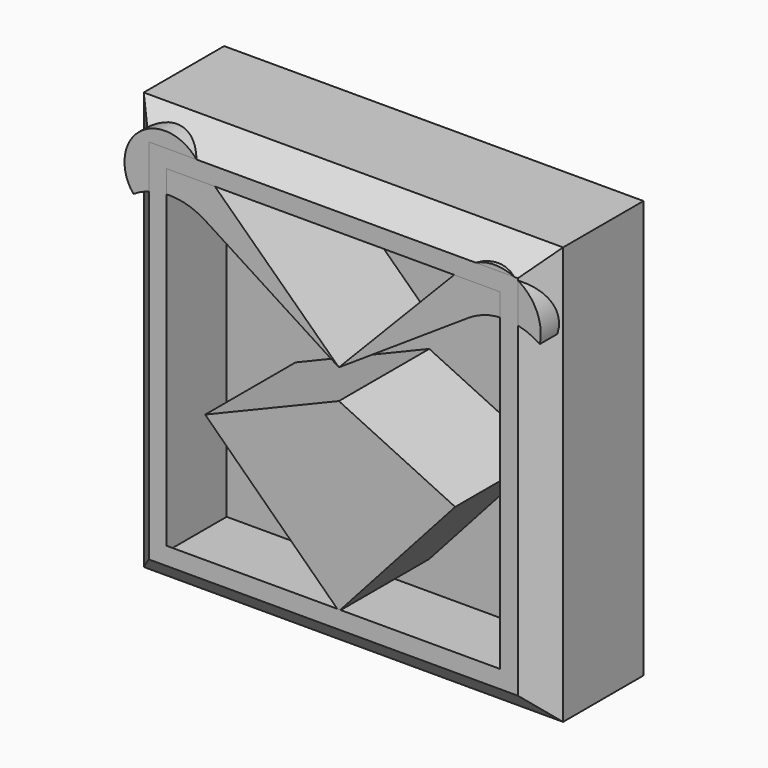
from build123d import *

# Parameters (mm, degrees)
F2_DEPTH = 25.4
F1_W     = 84.8106071353
F1_H     = 84.4905599952
F3_SIZE  = 5.08
F4_T     = -2.54


with BuildPart() as f2:
    # F0 (on Front) → F2 (new body)
    with BuildSketch(Plane.XZ):
        Polygon((23.5154349893, 0), (0, 11.1995805055), (-27.0433817059, 0), (0, -26.2091394757), align=None)
    extrude(amount=F2_DEPTH)


with BuildPart() as f2b:
    # F0 (on Front) → F2, piece 2 (new body)
    with BuildSketch(Plane.XZ):
        with BuildLine():
            Line((0, 17.1983804844), (-28.7676450394, 44.8085343447))
            ThreePointArc((-28.7676450394, 44.8085343447), (-40.2881972418, 46.0830542588), (-41.5627171559, 34.5625020564))
            ThreePointArc((-41.5627171559, 34.5625020564), (-34.3030494309, 36.6925224262), (-27.0433817059, 34.5625020564))
            Line((-27.0433817059, 34.5625020564), (0, 17.1983804844))
        make_face()
    extrude(amount=F2_DEPTH)


with BuildPart() as f2c:
    # F0 (on Front) → F2, piece 3 (new body)
    with BuildSketch(Plane.XZ):
        with BuildLine():
            Line((24.8967199784, 42.8875681139), (0, 17.1983804844))
            Line((0, 17.1983804844), (26.2432787567, 34.5625020564))
            ThreePointArc((26.2432787567, 34.5625020564), (33.4441801533, 36.7291108135), (40.6450815499, 34.5625020564))
            ThreePointArc((40.6450815499, 34.5625020564), (35.8939367202, 44.632819972), (24.8967199784, 42.8875681139))
        make_face()
    extrude(amount=F2_DEPTH)


with BuildPart() as f2d:
    # F1 (on Front) → F2, piece 4 (new body)
    with BuildSketch(Plane.XZ):
        with Locations((-1.1201389134, 7.6791383326)):
            Rectangle(F1_W, F1_H)
    extrude(amount=F2_DEPTH)

    # F3
    f3_edges = [f2d.edges().sort_by_distance(p)[0] for p in [
        (-43.525442, -25.4, 7.679138),
        (-1.120139, -25.4, 49.924418),
        (41.285165, -25.4, 7.679138),
        (-1.120139, -25.4, -34.566142),
    ]]
    chamfer(f3_edges, length=F3_SIZE)

    # F4
    f4_openings = [f2d.faces().sort_by_distance(p)[0] for p in [
        (-1.120139, -25.4, 7.679138),
    ]]
    offset(amount=F4_T, openings=f4_openings, kind=Kind.INTERSECTION)


solid = Compound([f2.part, f2b.part, f2c.part, f2d.part])
